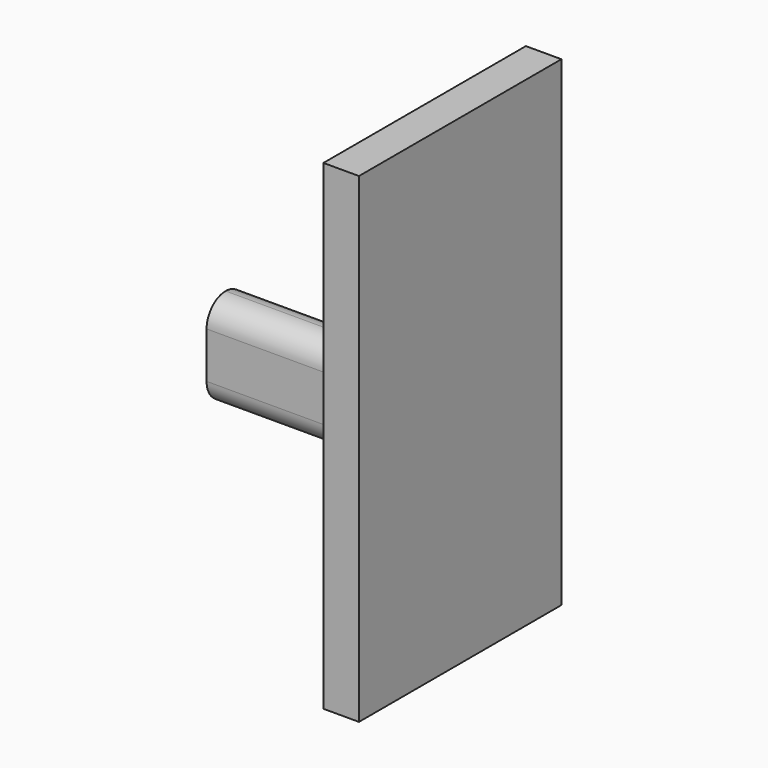
from build123d import *

# Parameters (mm, degrees)
F0_W     = 91.694
F0_H     = 50.1397587359
F1_DEPTH = 25.4
F2_R     = 12.69999
F4_D     = 6.35
F5_W     = 135.6123574078
F5_H     = 257.5739622116
F6_DEPTH = 19.05


# Not quite as in the source:
# - a fillet or chamfer is up to 0.001 mm smaller than in the source, because OpenCascade refuses the exact size


with BuildPart() as f1:
    # F0 (on Front) → F1 (new body)
    with BuildSketch(Plane.XZ):
        with Locations((-21.1153341503, 31.7568909377)):
            Rectangle(F0_W, F0_H)
    extrude(amount=F1_DEPTH)

    # F2 (radius 12.7 in the source; OpenCascade refuses exactly that, so slightly less here)
    f2_edges = [f1.edges().sort_by_distance(p)[0] for p in [
        (-21.115334, -25.4, 56.82677),
        (-21.115334, -25.4, 6.687012),
        (-21.115334, 0, 56.82677),
        (-21.115334, 0, 6.687012),
    ]]
    fillet(f2_edges, radius=F2_R)

    # F4 (through all)
    with Locations(Plane.YZ.offset(24.7316658497)):
        with Locations((-11.8228401989, 34.2414677143)):
            Hole(F4_D / 2)

    # F5 (on face) → F6 (join)
    with BuildSketch(Plane.YZ.offset(24.7316658497)):
        with Locations((6.0548242182, 38.2600277662)):
            Rectangle(F5_W, F5_H)
    extrude(amount=F6_DEPTH)


solid = f1.part
